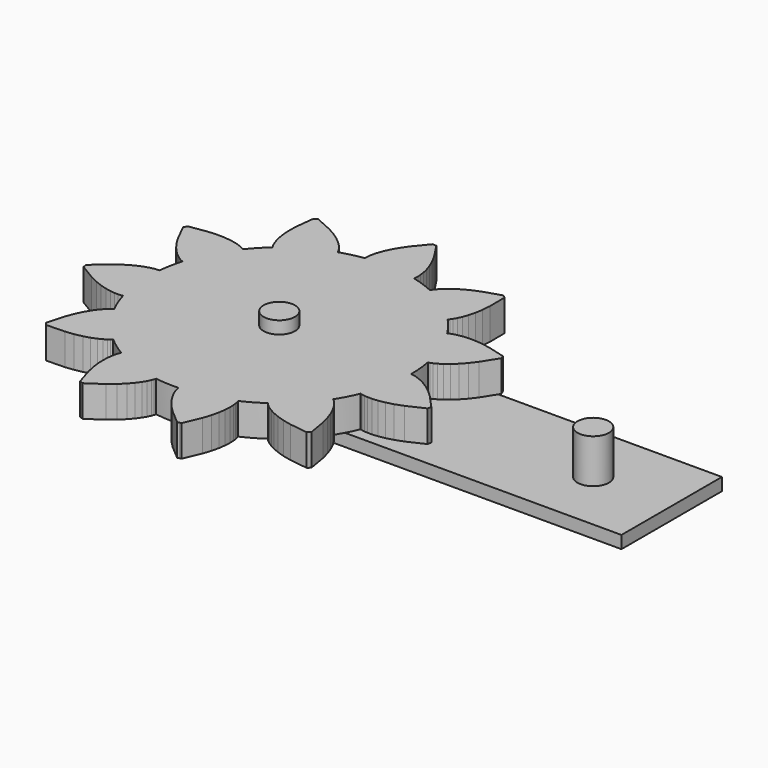
from build123d import *

# Parameters (mm, degrees)
F2_R     = 2.5
F3_DEPTH = 5
F4_W     = 75
F4_H     = 20
F4_R     = 2.5
F5_DEPTH = 2
F6_DEPTH = 7


with BuildPart() as f3:
    # F2 (on Top) → F3 (new body)
    with BuildSketch(Plane.XY):
        with BuildLine():
            Line((-28.6824429674, -0.0363065085), (-29, 0))
            ThreePointArc((-29, 0), (-29.0835825114, 1.8717583829), (-29.3336647089, 3.7286171213))
            Line((-29.3336647089, 3.7286171213), (-29.0275996118, 3.8207300292))
            Line((-29.0275996118, 3.8207300292), (-28.6591616705, 3.9758798267))
            Line((-28.6591616705, 3.9758798267), (-28.1641012201, 4.2369503744))
            Line((-28.1641012201, 4.2369503744), (-27.5591546847, 4.6266279875))
            Line((-27.5591546847, 4.6266279875), (-26.8639958507, 5.1653960163))
            Line((-26.8639958507, 5.1653960163), (-26.1009714476, 5.8712004949))
            Line((-26.1009714476, 5.8712004949), (-25.2948012678, 6.7591457746))
            Line((-25.2948012678, 6.7591457746), (-24.4722460972, 7.841223736))
            Line((-24.4722460972, 7.841223736), (-22.9022350115, 10.3301080648))
            ThreePointArc((-22.9022350115, 10.3301080648), (-22.9575731783, 10.4741181773), (-23.0136766754, 10.6178318607))
            ThreePointArc((-23.0136766754, 10.6178318607), (-23.0705439153, 10.7612450478), (-23.1281732883, 10.9043536799))
            Line((-23.1281732883, 10.9043536799), (-25.9732262329, 11.6561207673))
            Line((-25.9732262329, 11.6561207673), (-27.3125971913, 11.8875838503))
            Line((-27.3125971913, 11.8875838503), (-28.5076905728, 11.9881273136))
            Line((-28.5076905728, 11.9881273136), (-29.5470917874, 11.9847632286))
            Line((-29.5470917874, 11.9847632286), (-30.4230009301, 11.9053908973))
            Line((-30.4230009301, 11.9053908973), (-31.1312913018, 11.778372386))
            Line((-31.1312913018, 11.778372386), (-31.6715214883, 11.6321054177))
            Line((-31.6715214883, 11.6321054177), (-32.0469010546, 11.4945984817))
            Line((-32.0469010546, 11.4945984817), (-32.3336758105, 11.3534571666))
            ThreePointArc((-32.3336758105, 11.3534571666), (-33.4159388758, 12.8828924015), (-34.6302150342, 14.3097767315))
            Line((-34.6302150342, 14.3097767315), (-34.4225366877, 14.552738325))
            Line((-34.4225366877, 14.552738325), (-34.1964672814, 14.8824512299))
            Line((-34.1964672814, 14.8824512299), (-33.9211413228, 15.3697276371))
            Line((-33.9211413228, 15.3697276371), (-33.622903536, 16.0246040952))
            Line((-33.622903536, 16.0246040952), (-33.3293786985, 16.8536758431))
            Line((-33.3293786985, 16.8536758431), (-33.0690684341, 17.8599584913))
            Line((-33.0690684341, 17.8599584913), (-32.8709343841, 19.0427940998))
            Line((-32.8709343841, 19.0427940998), (-32.7639724545, 20.3978029075))
            Line((-32.7639724545, 20.3978029075), (-32.7887875402, 23.3403977186))
            ThreePointArc((-32.7887875402, 23.3403977186), (-32.9131987134, 23.4316286628), (-33.0380934619, 23.5221964661))
            ThreePointArc((-33.0380934619, 23.5221964661), (-33.163468251, 23.6120985654), (-33.2893195325, 23.7013324164))
            Line((-33.2893195325, 23.7013324164), (-36.0891663459, 22.7956073849))
            Line((-36.0891663459, 22.7956073849), (-37.3410552869, 22.2662079113))
            Line((-37.3410552869, 22.2662079113), (-38.4007897163, 21.7046741923))
            Line((-38.4007897163, 21.7046741923), (-39.2733708984, 21.1399014216))
            Line((-39.2733708984, 21.1399014216), (-39.9673206371, 20.5995769326))
            Line((-39.9673206371, 20.5995769326), (-40.4945010227, 20.1097914756))
            Line((-40.4945010227, 20.1097914756), (-40.8698936824, 19.6946733821))
            Line((-40.8698936824, 19.6946733821), (-41.1113412064, 19.3760496709))
            Line((-41.1113412064, 19.3760496709), (-41.276284727, 19.1022719024))
            ThreePointArc((-41.276284727, 19.1022719024), (-43.0136174697, 19.8037991088), (-44.8065634884, 20.3476833374))
            Line((-44.8065634884, 20.3476833374), (-44.7632083003, 20.6643550273))
            Line((-44.7632083003, 20.6643550273), (-44.7512828679, 21.0639495221))
            Line((-44.7512828679, 21.0639495221), (-44.7831054478, 21.6227249724))
            Line((-44.7831054478, 21.6227249724), (-44.8862647996, 22.3348816272))
            Line((-44.8862647996, 22.3348816272), (-45.0875660206, 23.1910326721))
            Line((-45.0875660206, 23.1910326721), (-45.4126165645, 24.1783058591))
            Line((-45.4126165645, 24.1783058591), (-45.8854248053, 25.2804898482))
            Line((-45.8854248053, 25.2804898482), (-46.5280157736, 26.4782237798))
            Line((-46.5280157736, 26.4782237798), (-48.1397784162, 28.9402760121))
            ThreePointArc((-48.1397784162, 28.9402760121), (-48.2937629274, 28.9497626079), (-48.4477957271, 28.9584298935))
            ThreePointArc((-48.4477957271, 28.9584298935), (-48.6018724558, 28.9662776236), (-48.7559887531, 28.9733055763))
            Line((-48.7559887531, 28.9733055763), (-50.6216978548, 26.6976497238))
            Line((-50.6216978548, 26.6976497238), (-51.388638885, 25.575468286))
            Line((-51.388638885, 25.575468286), (-51.9765561687, 24.5301403729))
            Line((-51.9765561687, 24.5301403729), (-52.4052789584, 23.5832702807))
            Line((-52.4052789584, 23.5832702807), (-52.6969451542, 22.7535428414))
            Line((-52.6969451542, 22.7535428414), (-52.8756395063, 22.0564938608))
            Line((-52.8756395063, 22.0564938608), (-52.967010122, 21.5043217037))
            Line((-52.967010122, 21.5043217037), (-52.9978677209, 21.1057419943))
            Line((-52.9978677209, 21.1057419943), (-52.9886116037, 20.7862502795))
            ThreePointArc((-52.9886116037, 20.7862502795), (-54.8294231535, 20.437139526), (-56.6317913399, 19.9253442536))
            Line((-56.6317913399, 19.9253442536), (-56.766524276, 20.2151850158))
            Line((-56.766524276, 20.2151850158), (-56.9725290583, 20.5577926717))
            Line((-56.9725290583, 20.5577926717), (-57.3013967322, 21.0106599077))
            Line((-57.3013967322, 21.0106599077), (-57.7732008573, 21.5539920532))
            Line((-57.7732008573, 21.5539920532), (-58.4054164215, 22.1654004877))
            Line((-58.4054164215, 22.1654004877), (-59.2126265228, 22.8202119524))
            Line((-59.2126265228, 22.8202119524), (-60.2062637786, 23.4918086933))
            Line((-60.2062637786, 23.4918086933), (-61.3943895526, 24.1519956882))
            Line((-61.3943895526, 24.1519956882), (-64.0813765014, 25.351821154))
            ThreePointArc((-64.0813765014, 25.351821154), (-64.2160453563, 25.2765514742), (-64.3503118816, 25.2005664401))
            ThreePointArc((-64.3503118816, 25.2005664401), (-64.4841722772, 25.1238682023), (-64.6176227548, 25.0464589313))
            Line((-64.6176227548, 25.0464589313), (-64.9568446875, 22.1233769121))
            Line((-64.9568446875, 22.1233769121), (-64.9953394487, 20.7646981875))
            Line((-64.9953394487, 20.7646981875), (-64.9247800033, 19.5674603067))
            Line((-64.9247800033, 19.5674603067), (-64.7735279441, 18.539117457))
            Line((-64.7735279441, 18.539117457), (-64.5703086406, 17.6834196669))
            Line((-64.5703086406, 17.6834196669), (-64.3437827649, 17.0004152889))
            Line((-64.3437827649, 17.0004152889), (-64.1221218118, 16.4864998266))
            Line((-64.1221218118, 16.4864998266), (-63.932592416, 16.1345103604))
            Line((-63.932592416, 16.1345103604), (-63.7520754129, 15.8707410614))
            ThreePointArc((-63.7520754129, 15.8707410614), (-65.1119211092, 14.5818325456), (-66.351472299, 13.176849155))
            Line((-66.351472299, 13.176849155), (-66.6215166041, 13.3478365954))
            Line((-66.6215166041, 13.3478365954), (-66.9800465381, 13.5246819025))
            Line((-66.9800465381, 13.5246819025), (-67.5015461434, 13.7278587766))
            Line((-67.5015461434, 13.7278587766), (-68.1922005657, 13.9298622956))
            Line((-68.1922005657, 13.9298622956), (-69.0546064984, 14.1024102617))
            Line((-69.0546064984, 14.1024102617), (-70.0876926534, 14.2168619907))
            Line((-70.0876926534, 14.2168619907), (-71.2866861162, 14.2446442634))
            Line((-71.2866861162, 14.2446442634), (-72.6431251577, 14.1576796155))
            Line((-72.6431251577, 14.1576796155), (-75.5522370416, 13.7143422069))
            ThreePointArc((-75.5522370416, 13.7143422069), (-75.6248338304, 13.578213843), (-75.6967054081, 13.4417012007))
            ThreePointArc((-75.6967054081, 13.4417012007), (-75.7678497408, 13.3048081434), (-75.8382648151, 13.1675385455))
            Line((-75.8382648151, 13.1675385455), (-74.543299012, 10.525088247))
            Line((-74.543299012, 10.525088247), (-73.8411256896, 9.3612831308))
            Line((-73.8411256896, 9.3612831308), (-73.1344916402, 8.3922498502))
            Line((-73.1344916402, 8.3922498502), (-72.4512861922, 7.6089258319))
            Line((-72.4512861922, 7.6089258319), (-71.8177020825, 6.9989356933))
            Line((-71.8177020825, 6.9989356933), (-71.257876344, 6.5468249819))
            Line((-71.257876344, 6.5468249819), (-70.7935596085, 6.2343307426))
            Line((-70.7935596085, 6.2343307426), (-70.4438174619, 6.0406856882))
            Line((-70.4438174619, 6.0406856882), (-70.1493524459, 5.9163836937))
            ThreePointArc((-70.1493524459, 5.9163836937), (-70.5964908885, 4.0968967623), (-70.8796763372, 2.2447975529))
            Line((-70.8796763372, 2.2447975529), (-71.1992948525, 2.2426443673))
            Line((-71.1992948525, 2.2426443673), (-71.5965192174, 2.1975801901))
            Line((-71.5965192174, 2.1975801901), (-72.145078314, 2.0865594804))
            Line((-72.145078314, 2.0865594804), (-72.8353051345, 1.8830996829))
            Line((-72.8353051345, 1.8830996829), (-73.6540936455, 1.5620044205))
            Line((-73.6540936455, 1.5620044205), (-74.5850582994, 1.0997587985))
            Line((-74.5850582994, 1.0997587985), (-75.6087360164, 0.4749059277))
            Line((-75.6087360164, 0.4749059277), (-76.7028285138, -0.3315997018))
            Line((-76.7028285138, -0.3315997018), (-78.9104428646, -2.2773434899))
            ThreePointArc((-78.9104428646, -2.2773434899), (-78.8979186197, -2.4311107442), (-78.8845765318, -2.5848091954))
            ThreePointArc((-78.8845765318, -2.5848091954), (-78.8704169787, -2.7384344936), (-78.855440361, -2.8919822912))
            Line((-78.855440361, -2.8919822912), (-76.3374293148, -4.4148415698))
            Line((-76.3374293148, -4.4148415698), (-75.1175229773, -5.0142731762))
            Line((-75.1175229773, -5.0142731762), (-73.9991656419, -5.4474406369))
            Line((-73.9991656419, -5.4474406369), (-73.0009197075, -5.7370459827))
            Line((-73.0009197075, -5.7370459827), (-72.1381292697, -5.9076609109))
            Line((-72.1381292697, -5.9076609109), (-71.4227443848, -5.9853359991))
            Line((-71.4227443848, -5.9853359991), (-70.8631891497, -5.9971943025))
            Line((-70.8631891497, -5.9971943025), (-70.4642749128, -5.9710140086))
            Line((-70.4642749128, -5.9710140086), (-70.1493524459, -5.9163836937))
            ThreePointArc((-70.1493524459, -5.9163836937), (-69.5418203385, -7.6887747957), (-68.7787306671, -9.3999614113))
            Line((-68.7787306671, -9.3999614113), (-69.0464467722, -9.5745716016))
            Line((-69.0464467722, -9.5745716016), (-69.3562496389, -9.8272377053))
            Line((-69.3562496389, -9.8272377053), (-69.7577045896, -10.217207708))
            Line((-69.7577045896, -10.217207708), (-70.2283616696, -10.7615337739))
            Line((-70.2283616696, -10.7615337739), (-70.743573192, -11.4743267876))
            Line((-70.743573192, -11.4743267876), (-71.2768416451, -12.3665100416))
            Line((-71.2768416451, -12.3665100416), (-71.8001931742, -13.4456116845))
            Line((-71.8001931742, -13.4456116845), (-72.28457249, -14.7155984567))
            Line((-72.28457249, -14.7155984567), (-73.0897873495, -17.5459887197))
            ThreePointArc((-73.0897873495, -17.5459887197), (-72.9961184302, -17.6685748476), (-72.9017986954, -17.7906609354))
            ThreePointArc((-72.9017986954, -17.7906609354), (-72.8068308145, -17.9122435278), (-72.7112174751, -18.0333191841))
            Line((-72.7112174751, -18.0333191841), (-69.7696119016, -17.9530903819))
            Line((-69.7696119016, -17.9530903819), (-68.4192841917, -17.797833179))
            Line((-68.4192841917, -17.797833179), (-67.2442741223, -17.5576072115))
            Line((-67.2442741223, -17.5576072115), (-66.2479237324, -17.2615462339))
            Line((-66.2479237324, -17.2615462339), (-65.4298568343, -16.9386169173))
            Line((-65.4298568343, -16.9386169173), (-64.7860424494, -16.6171950908))
            Line((-64.7860424494, -16.6171950908), (-64.3089035482, -16.3246525307))
            Line((-64.3089035482, -16.3246525307), (-63.9874696726, -16.0869589469))
            Line((-63.9874696726, -16.0869589469), (-63.7520754129, -15.8707410614))
            ThreePointArc((-63.7520754129, -15.8707410614), (-62.2827599069, -17.0333146824), (-60.7156706943, -18.0602990444))
            Line((-60.7156706943, -18.0602990444), (-60.8464864175, -18.3519287377))
            Line((-60.8464864175, -18.3519287377), (-60.9705075647, -18.7319770652))
            Line((-60.9705075647, -18.7319770652), (-61.0973992593, -19.2770836404))
            Line((-61.0973992593, -19.2770836404), (-61.1990563013, -19.9894562948))
            Line((-61.1990563013, -19.9894562948), (-61.2471148171, -20.8676403144))
            Line((-61.2471148171, -20.8676403144), (-61.2133781034, -21.9064993212))
            Line((-61.2133781034, -21.9064993212), (-61.0702430319, -23.097242589))
            Line((-61.0702430319, -23.097242589), (-60.7911221559, -24.4274986771))
            Line((-60.7911221559, -24.4274986771), (-59.9382874956, -27.243906505))
            ThreePointArc((-59.9382874956, -27.243906505), (-59.7932131219, -27.296391277), (-59.6478615895, -27.3481035311))
            ThreePointArc((-59.6478615895, -27.3481035311), (-59.502237012, -27.3990418038), (-59.3563435107, -27.4492046535))
            Line((-59.3563435107, -27.4492046535), (-56.925082395, -25.7913598483))
            Line((-56.925082395, -25.7913598483), (-55.8730528196, -24.9307069009))
            Line((-55.8730528196, -24.9307069009), (-55.0144474111, -24.0933575527))
            Line((-55.0144474111, -24.0933575527), (-54.3363267747, -23.3056275201))
            Line((-54.3363267747, -23.3056275201), (-53.8227138762, -22.5916817351))
            Line((-53.8227138762, -22.5916817351), (-53.4548765094, -21.9732121526))
            Line((-53.4548765094, -21.9732121526), (-53.211642172, -21.4691489249))
            Line((-53.211642172, -21.4691489249), (-53.069741642, -21.0954080845))
            Line((-53.069741642, -21.0954080845), (-52.9886116037, -20.7862502795))
            ThreePointArc((-52.9886116037, -20.7862502795), (-51.1240099907, -20.9698975091), (-49.2504609894, -20.9866193388))
            Line((-49.2504609894, -20.9866193388), (-49.2028432629, -21.3026781682))
            Line((-49.2028432629, -21.3026781682), (-49.1017068527, -21.6894460607))
            Line((-49.1017068527, -21.6894460607), (-48.9137480746, -22.2166217224))
            Line((-48.9137480746, -22.2166217224), (-48.6141296862, -22.8708676808))
            Line((-48.6141296862, -22.8708676808), (-48.1797769561, -23.6356254851))
            Line((-48.1797769561, -23.6356254851), (-47.5897462439, -24.4913298502))
            Line((-47.5897462439, -24.4913298502), (-46.8255689456, -25.4156621688))
            Line((-46.8255689456, -25.4156621688), (-45.8715667837, -26.3838406639))
            Line((-45.8715667837, -26.3838406639), (-43.6314515824, -28.2920764712))
            ThreePointArc((-43.6314515824, -28.2920764712), (-43.481031843, -28.2577963431), (-43.3307965975, -28.2227164882))
            ThreePointArc((-43.3307965975, -28.2227164882), (-43.1807500978, -28.1868378995), (-43.0308965904, -28.1501615922))
            Line((-43.0308965904, -28.1501615922), (-41.8818881583, -25.4410547958))
            Line((-41.8818881583, -25.4410547958), (-41.4621686744, -24.1482573337))
            Line((-41.4621686744, -24.1482573337), (-41.1925690772, -22.9796371064))
            Line((-41.1925690772, -22.9796371064), (-41.0479767049, -21.9503367383))
            Line((-41.0479767049, -21.9503367383), (-41.0018862724, -21.0720472272))
            Line((-41.0018862724, -21.0720472272), (-41.0268116887, -20.3528896113))
            Line((-41.0268116887, -20.3528896113), (-41.0947070986, -19.7973422292))
            Line((-41.0947070986, -19.7973422292), (-41.1773923299, -19.4062142083))
            Line((-41.1773923299, -19.4062142083), (-41.276284727, -19.1022719024))
            ThreePointArc((-41.276284727, -19.1022719024), (-39.6083948444, -18.2486860428), (-38.0232246244, -17.2498362775))
            Line((-38.0232246244, -17.2498362775), (-37.8122917398, -17.4899777977))
            Line((-37.8122917398, -17.4899777977), (-37.5181078679, -17.7606691823))
            Line((-37.5181078679, -17.7606691823), (-37.0749742011, -18.1025393826))
            Line((-37.0749742011, -18.1025393826), (-36.4692071036, -18.490940176))
            Line((-36.4692071036, -18.490940176), (-35.6903470505, -18.8994665656))
            Line((-35.6903470505, -18.8994665656), (-34.7313529219, -19.3003361992))
            Line((-34.7313529219, -19.3003361992), (-33.5887542896, -19.6647885886))
            Line((-33.5887542896, -19.6647885886), (-32.2627597875, -19.9634996593))
            Line((-32.2627597875, -19.9634996593), (-29.3465847938, -20.3577120601))
            ThreePointArc((-29.3465847938, -20.3577120601), (-29.2385768931, -20.2475507303), (-29.1311565634, -20.1368163725))
            ThreePointArc((-29.1311565634, -20.1368163725), (-29.0243268451, -20.0255121207), (-28.9180907613, -19.9136411249))
            Line((-28.9180907613, -19.9136411249), (-29.4161370715, -17.0133946036))
            Line((-29.4161370715, -17.0133946036), (-29.7619856496, -15.6989066865))
            Line((-29.7619856496, -15.6989066865), (-30.166987831, -14.5700442451))
            Line((-30.166987831, -14.5700442451), (-30.6018307794, -13.6259691358))
            Line((-30.6018307794, -13.6259691358), (-31.0378961994, -12.8621866126))
            Line((-31.0378961994, -12.8621866126), (-31.4476707553, -12.2706684251))
            Line((-31.4476707553, -12.2706684251), (-31.8051395995, -11.8400192571))
            Line((-31.8051395995, -11.8400192571), (-32.0861586154, -11.5556844388))
            Line((-32.0861586154, -11.5556844388), (-32.3336758105, -11.3534571666))
            ThreePointArc((-32.3336758105, -11.3534571666), (-31.3920409114, -9.7336456971), (-30.5985298173, -8.0363520797))
            Line((-30.5985298173, -8.0363520797), (-30.2912514752, -8.1243330548))
            Line((-30.2912514752, -8.1243330548), (-29.8974214422, -8.1930053293))
            Line((-29.8974214422, -8.1930053293), (-29.3398046949, -8.2410286953))
            Line((-29.3398046949, -8.2410286953), (-28.6202156616, -8.2402698161))
            Line((-28.6202156616, -8.2402698161), (-27.7441308491, -8.1628605488))
            Line((-27.7441308491, -8.1628605488), (-26.720647164, -7.9816221747))
            Line((-26.720647164, -7.9816221747), (-25.5623941904, -7.6704835762))
            Line((-25.5623941904, -7.6704835762), (-24.2854012335, -7.2048885682))
            Line((-24.2854012335, -7.2048885682), (-21.6190314031, -5.9599179106))
            ThreePointArc((-21.6190314031, -5.9599179106), (-21.5877270864, -5.8088508229), (-21.5572268683, -5.6576193385))
            ThreePointArc((-21.5572268683, -5.6576193385), (-21.527531612, -5.5062277371), (-21.4986421578, -5.3546803035))
            Line((-21.4986421578, -5.3546803035), (-23.4856170258, -3.1841018357))
            Line((-23.4856170258, -3.1841018357), (-24.4872291861, -2.2652640895))
            Line((-24.4872291861, -2.2652640895), (-25.4382478151, -1.5345652831))
            Line((-25.4382478151, -1.5345652831), (-26.3144665205, -0.9754526092))
            Line((-26.3144665205, -0.9754526092), (-27.0942401034, -0.5686726284))
            Line((-27.0942401034, -0.5686726284), (-27.7587632726, -0.2925967142))
            Line((-27.7587632726, -0.2925967142), (-28.2923117189, -0.1235738284))
            Line((-28.2923117189, -0.1235738284), (-28.6824429674, -0.0363065085))
        make_face()
        with Locations((-50, 0)):
            Circle(F2_R, mode=Mode.SUBTRACT)
    extrude(amount=F3_DEPTH)


with BuildPart() as f5:
    # F4 (on Top) → F5 (new body)
    with BuildSketch(Plane.XY):
        with Locations((-25, 0)):
            Rectangle(F4_W, F4_H)
        with Locations((-50, 0)):
            Circle(F4_R, mode=Mode.SUBTRACT)
        Circle(F4_R, mode=Mode.SUBTRACT)
        with Locations((-50, 0)):
            Circle(F4_R)
        Circle(F4_R)
    extrude(amount=-F5_DEPTH)

    # F4 (on Top) → F6 (join)
    with BuildSketch(Plane.XY):
        with Locations((-50, 0)):
            Circle(F4_R)
        Circle(F4_R)
    extrude(amount=F6_DEPTH)


solid = Compound([f3.part, f5.part])
